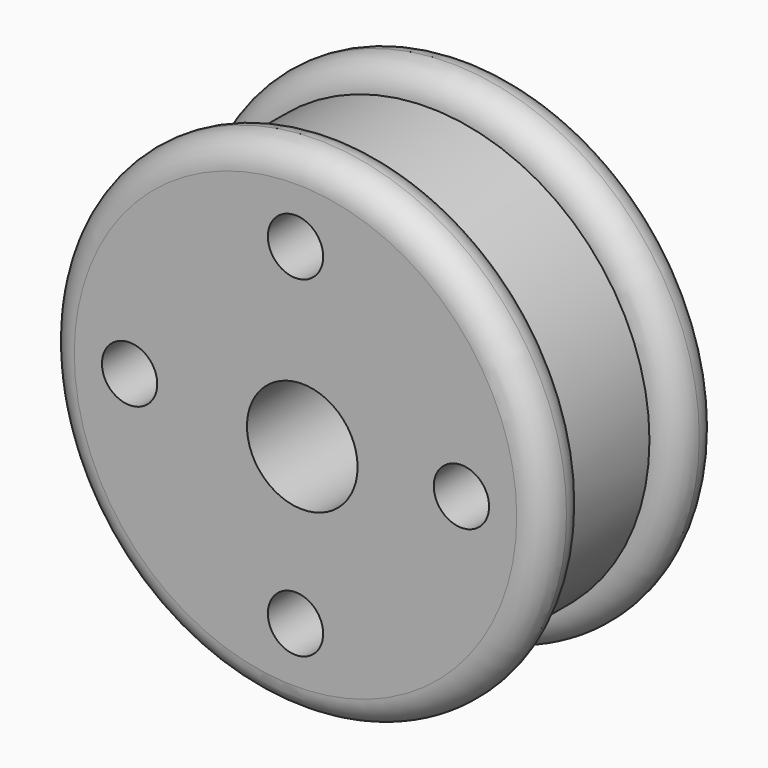
from build123d import *

# Parameters (mm, degrees)
F0_R      = 28.575
F1_DEPTH  = 6.35
F2_R      = 25.4
F3_DEPTH  = 12.7
F4_R      = 28.575
F5_DEPTH  = 6.35
F6_R      = 3.175
F7_DEPTH  = 25.401
F8_R      = 3.17499
F9_R      = 6.35
F10_DEPTH = 25.401


# Not quite as in the source:
# - a fillet or chamfer is up to 0.001 mm smaller than in the source, because OpenCascade refuses the exact size


with BuildPart() as f1:
    # F0 (on Front) → F1 (new body)
    with BuildSketch(Plane.XZ):
        Circle(F0_R)
    extrude(amount=F1_DEPTH)

    # F2 (on face) → F3 (join)
    with BuildSketch(Plane.XZ.offset(6.35)):
        Circle(F2_R)
    extrude(amount=F3_DEPTH)

    # F4 (on face) → F5 (join)
    with BuildSketch(Plane.XZ.offset(19.05)):
        Circle(F4_R)
    extrude(amount=F5_DEPTH)

    # F6 (on face) → F7 (cut, through all)
    with BuildSketch(Plane.XZ.offset(25.4)):
        with Locations((0, 19.05)):
            Circle(F6_R)
        with Locations((19.05, 0)):
            Circle(F6_R)
        with Locations((0, -19.05)):
            Circle(F6_R)
        with Locations((-19.05, 0)):
            Circle(F6_R)
    extrude(amount=-F7_DEPTH, mode=Mode.SUBTRACT)

    # F8 (radius 3.175 in the source; OpenCascade refuses exactly that, so slightly less here)
    f8_edges = [f1.edges().sort_by_distance(p)[0] for p in [
        (-28.575, -25.4, 0),
        (-28.575, -19.05, 0),
        (-28.575, -6.35, 0),
        (-28.575, 0, 0),
    ]]
    fillet(f8_edges, radius=F8_R)

    # F9 (on face) → F10 (cut, through all)
    with BuildSketch(Plane.XZ.offset(25.4)):
        with Locations((0.7773180259, -0.9165679221)):
            Circle(F9_R)
    extrude(amount=-F10_DEPTH, mode=Mode.SUBTRACT)


solid = f1.part
